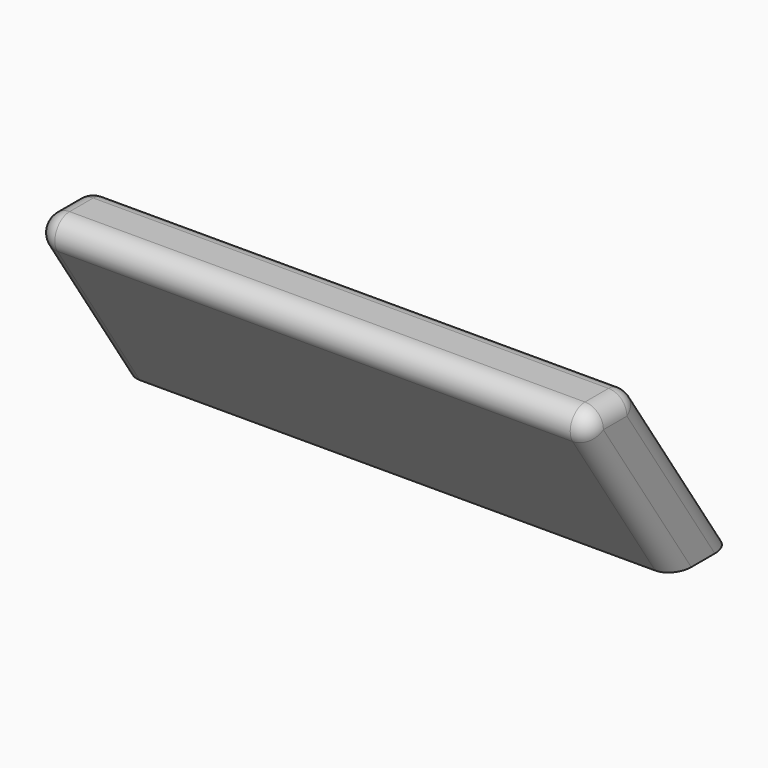
from build123d import *

# Parameters (mm, degrees)
F1_DEPTH = 75
F2_F1_R  = 5
F2_F2_R  = 5
F2_F3_R  = 5
F2_F4_R  = 5


# Not quite as in the source:
# - a feature of the source that left no trace in its solid (it failed there, or was rolled back) is left out


with BuildPart() as f1:
    # F0 (on Right) → F1 (new body, symmetric)
    with BuildSketch(Plane.YZ):
        Polygon((-15.2537021786, 50), (17.912545725, 0), (37.912545725, 0), (4.7462978214, 50), align=None)
    extrude(amount=F1_DEPTH, both=True)

    # F2: fillet of radius 5 on 4 edges, made by hand

    # F2_f1
    f2_f1_edges = [f1.edges().sort_by_distance(p)[0] for p in [
        (0, -15.2537021786, 50),
    ]]
    fillet(f2_f1_edges, radius=F2_F1_R)

    # F2_f2
    f2_f2_edges = [f1.edges().sort_by_distance(p)[0] for p in [
        (0, 4.7462978214, 50),
    ]]
    fillet(f2_f2_edges, radius=F2_F2_R)

    # F2_f3
    f2_f3_edges = [f1.edges().sort_by_distance(p)[0] for p in [
        (-75, -1.9370773882, 50),
    ]]
    fillet(f2_f3_edges, radius=F2_F3_R)

    # F2_f4
    f2_f4_edges = [f1.edges().sort_by_distance(p)[0] for p in [
        (75, -1.9370773882, 50),
    ]]
    fillet(f2_f4_edges, radius=F2_F4_R)


solid = f1.part
